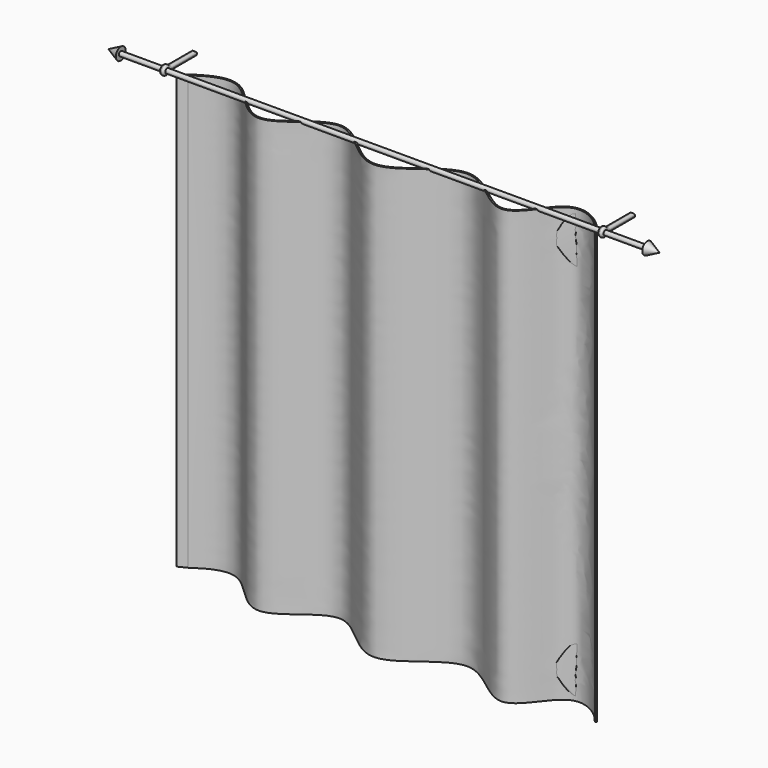
from build123d import *

# Parameters (mm, degrees)
F3_R     = 7.5
F4_DEPTH = 15
F5_R     = 7
F8_DEPTH = 1400


# Not quite as in the source:
# - ends of sketch curves that miss each other by under 0.0002 mm in the source are joined
# - the dataset's text gives a spline's control points without its knots; the knots are read off the source's solid


with BuildPart() as f1:
    # F0 (on Front) → F1 (revolve)
    with BuildSketch(Plane.XZ):
        Polygon((-850, 20), (-890, 0), (890, 0), (850, 20), (850, 7.5), (-850, 7.5), align=None)
    revolve(axis=Axis((0, 0, 0), (-1, 0, 0)))


with BuildPart() as f4:
    # F3 (on offset) → F4 (new body)
    with BuildSketch(Plane.YZ.offset(700)):
        with BuildLine():
            Line((120, 7.5), (12.9903810568, 7.5))
            ThreePointArc((12.9903810568, 7.5), (-15, 0), (12.9903810568, -7.5))
            Line((12.9903810568, -7.5), (120, -7.5))
            Line((120, -7.5), (120, 7.5))
        make_face()
        Circle(F3_R, mode=Mode.SUBTRACT)
    extrude(amount=F4_DEPTH)

    # F5
    f5_edges = [f4.edges().sort_by_distance(p)[0] for p in [
        (707.5, 120, 7.5),
        (707.5, 12.990381, 7.5),
        (700, 66.495191, 7.5),
        (715, 66.495191, 7.5),
        (707.5, 12.990381, -7.5),
        (700, -15, 0),
        (715, -15, 0),
        (707.5, 120, -7.5),
        (700, 66.495191, -7.5),
        (715, 66.495191, -7.5),
    ]]
    fillet(f5_edges, radius=F5_R)


with BuildPart() as f6_1:
    # F6: instance of F4
    add(f4.part.mirror(Plane.YZ))


with BuildPart() as f8:
    # F7 (on Top) → F8 (new body)
    with BuildSketch(Plane.XY):
        with BuildLine():
            add(Edge.make_bspline(
                [(-670.6937551498, 0), (-614.3739529849, 43.1276240513), (-503.935100688, 108.8308960068), (-362.2673319574, -141.7782707313), (-166.2526515003, 141.5498224049), (22.0472697916, -177.7934265192), (238.5955784254, 142.9164890413), (441.9004095898, -150.6435928961), (540.9393764759, 113.8261303534), (657.7247773689, 40.7478963714), (687.0885491371, 0)],
                knots=[0, 0, 0, 0, 0.1167059495, 0.2396336092, 0.3697119181, 0.504489529, 0.6451028195, 0.7761697664, 0.8935284317, 1, 1, 1, 1], degree=3))
            Line((-670.6937551498, 0), (-643.763785974, 13.6410482552))
            add(Edge.make_bspline(
                [(-643.763785974, 13.6410482552), (-636.913039698, 18.4570202201), (-622.8116029597, 27.8819588686), (-601.835543085, 39.8472046621), (-580.8970297945, 49.0102192481), (-563.9802501877, 53.6015366481), (-550.7924221753, 55.2006128136), (-541.0678849864, 55.3066074937), (-531.4927513032, 54.259609341), (-523.6156599952, 52.3702724168), (-517.3569747691, 50.2070864292), (-512.6867218869, 48.2491445642), (-508.0117992724, 45.9350459268), (-501.7596420883, 42.4005152749), (-493.9211466123, 37.2019668625), (-484.4899357328, 29.9215322439), (-475.0408732434, 21.8176835289), (-462.4154959996, 10.2112084592), (-446.5650151802, -5.239923565), (-430.5158822065, -20.4646579487), (-417.4503350768, -31.6254561731), (-407.5009759804, -39.264870881), (-397.3576903794, -45.9470072709), (-386.9689347873, -51.4350318847), (-378.0626806236, -54.7984958048), (-370.7734333609, -56.6194547196), (-365.2254024954, -57.5118147501), (-360.5407224445, -57.8299001173), (-356.7571596564, -57.8102668966), (-352.9714098517, -57.6059984282), (-348.2424308865, -57.0205733142), (-340.6901447793, -55.4369622065), (-331.2816799091, -52.352352747), (-320.0236402265, -47.1935972314), (-308.7691812475, -40.8541260767), (-297.4988233468, -33.5924104819), (-286.2032650196, -25.6588137615), (-271.1087613436, -14.5151486282), (-252.191143483, -0.142740191), (-233.3030507696, 13.1657275771), (-218.3158678651, 22.1834426885), (-207.1749186377, 27.8900885994), (-196.175911243, 32.3073460769), (-187.1651444335, 34.7352860958), (-180.0617413253, 35.8316499626), (-175.6643659457, 36.1464262602), (-172.1698702327, 36.1652394346), (-168.6873732305, 36.0240411136), (-164.3186611921, 35.549956619), (-159.0502972196, 34.5270893651), (-151.9825660211, 32.5852115468), (-143.0644779709, 29.1275415894), (-132.2436342222, 23.5228691932), (-117.6891114969, 14.401380201), (-99.3102972555, 0.4904906162), (-77.0246789272, -18.2786131316), (-58.2332577732, -34.0220632618), (-43.012491741, -45.7071731766), (-31.4799807719, -53.7725884064), (-19.8020341734, -60.8927964534), (-7.9431652974, -66.8131627408), (2.1221885969, -70.5220483502), (10.2973244286, -72.6074092029), (16.4896351805, -73.6912527844), (21.6989124907, -74.1620866053), (25.890357465, -74.2586097388), (30.0769044192, -74.1701029531), (35.304455582, -73.7258056175), (43.6451097686, -72.3525018059), (54.0199363775, -69.4888468875), (66.3931050228, -64.5038198354), (78.7122357244, -58.2331567927), (90.9984421726, -50.9233215282), (103.2671912498, -42.8117191421), (119.6138193679, -31.2382536138), (140.0357688863, -15.9295393415), (164.4984950231, 1.935332908), (184.7714630248, 14.8533931425), (200.8368775522, 23.0919904282), (212.780022253, 28.0049222573), (222.6206443148, 30.8722205887), (230.4179320306, 32.336378693), (236.2295867624, 32.9977474251), (241.0442382147, 33.1671740352), (244.8840932803, 33.0615991942), (248.7354882724, 32.7966852748), (253.5659590208, 32.1755307596), (261.3334546625, 30.5948681413), (271.1106516001, 27.5799881614), (282.9179121968, 22.5102470797), (294.7539358949, 16.2189931957), (310.5158856967, 6.5266408618), (330.0832382885, -7.4080889802), (349.2692670927, -22.0731226427), (364.3133942811, -33.226916937), (375.435094448, -41.0506433385), (386.3938503105, -48.0797792734), (397.2012748421, -54.058358024), (407.8853517187, -58.7191517001), (416.7236170186, -61.2582920899), (423.7681966191, -62.3043958063), (428.155532052, -62.5045421958), (431.6485467186, -62.3672958008), (435.1260281475, -62.0220765234), (439.3879361412, -61.2090209039), (444.3615208454, -59.6754592837), (450.7993285941, -56.9566056159), (458.4994777713, -52.4233909767), (467.2909074427, -45.5203161881), (475.7524534834, -37.4457534801), (483.983143576, -28.4658227454), (494.757346215, -15.6297969749), (508.0231877001, 1.3900534297), (521.3889393854, 17.9677676889), (532.300580103, 29.8986613037), (540.6184128273, 37.9145016088), (547.6731812707, 43.6002928254), (553.3920497432, 47.4322226329), (556.9976870507, 49.5063049507), (559.9022257026, 50.9613448303), (562.8197155458, 52.2754644668), (566.5222584039, 53.6679987047), (571.0467434202, 54.9540652287), (577.1837700139, 56.1737878851), (585.0379816061, 56.8007883765), (594.6979161308, 56.2021711556), (604.5116823025, 54.3342447701), (617.6745431072, 50.269448945), (634.0178531075, 42.4751040133), (652.6212039978, 29.6325248002), (669.4069118431, 14.2183195432), (678.8637644961, 2.8611485143), (683.0320714182, -2.9231812321)],
                knots=[0.0167269107, 0.0167269107, 0.0167269107, 0.0167269107, 0.03125, 0.046875, 0.0625, 0.078125, 0.0859375, 0.09375, 0.1015625, 0.109375, 0.11328125, 0.1171875, 0.12109375, 0.125, 0.1328125, 0.140625, 0.1484375, 0.15625, 0.171875, 0.1875, 0.1953125, 0.203125, 0.2109375, 0.21875, 0.2265625, 0.23046875, 0.234375, 0.23828125, 0.240234375, 0.2421875, 0.24609375, 0.25, 0.2578125, 0.265625, 0.2734375, 0.28125, 0.2890625, 0.296875, 0.3125, 0.328125, 0.3359375, 0.34375, 0.3515625, 0.359375, 0.36328125, 0.3671875, 0.369140625, 0.37109375, 0.375, 0.37890625, 0.3828125, 0.390625, 0.3984375, 0.40625, 0.421875, 0.4375, 0.453125, 0.4609375, 0.46875, 0.4765625, 0.484375, 0.4921875, 0.49609375, 0.5, 0.50390625, 0.505859375, 0.5078125, 0.51171875, 0.515625, 0.5234375, 0.53125, 0.5390625, 0.546875, 0.5546875, 0.5625, 0.578125, 0.59375, 0.609375, 0.6171875, 0.625, 0.6328125, 0.63671875, 0.640625, 0.64453125, 0.646484375, 0.6484375, 0.65234375, 0.65625, 0.6640625, 0.671875, 0.6796875, 0.6875, 0.703125, 0.71875, 0.7265625, 0.734375, 0.7421875, 0.75, 0.7578125, 0.765625, 0.76953125, 0.7734375, 0.775390625, 0.77734375, 0.78125, 0.78515625, 0.7890625, 0.796875, 0.8046875, 0.8125, 0.8203125, 0.828125, 0.84375, 0.859375, 0.8671875, 0.875, 0.8828125, 0.88671875, 0.890625, 0.892578125, 0.89453125, 0.8984375, 0.90234375, 0.90625, 0.9140625, 0.921875, 0.9296875, 0.9375, 0.953125, 0.96875, 0.984375, 1, 1, 1, 1], degree=3))
            Line((683.0320714182, -2.9231812321), (687.0885491371, 0))
        make_face()
    extrude(amount=-F8_DEPTH)


solid = Compound([f1.part, f4.part, f6_1.part, f8.part])
